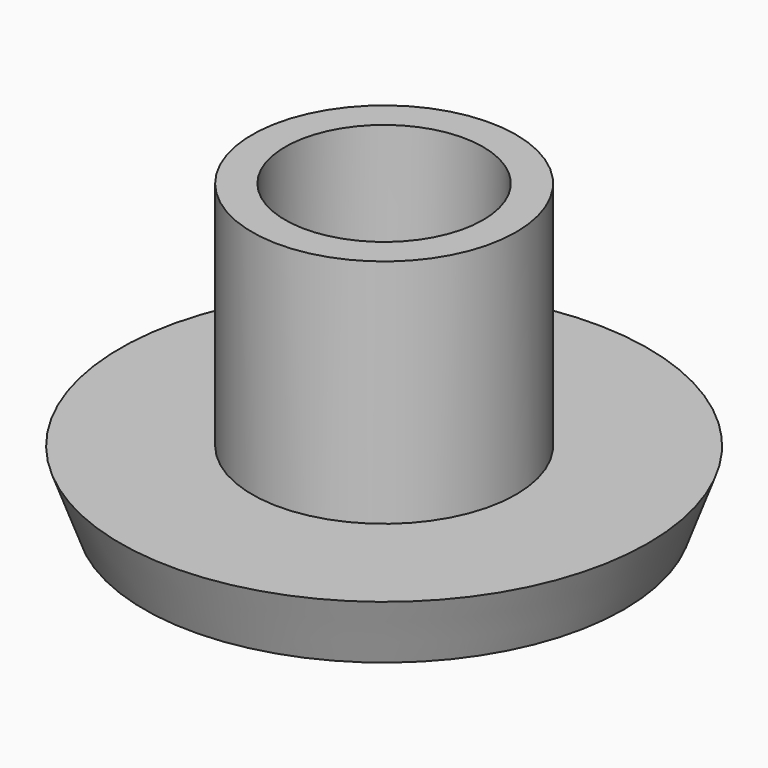
from build123d import *

# Parameters (mm, degrees)
F0_R     = 4
F0_R_2   = 3
F1_DEPTH = 7
F0_R_3   = 8
F2_DEPTH = 2
F3_SIZE2 = 0.72793
F3_SIZE  = 1.99999
F4_DEPTH = 2


# Not quite as in the source:
# - a fillet or chamfer is up to 0.001 mm smaller than in the source, because OpenCascade refuses the exact size


with BuildPart() as f1:
    # F0 (on Top) → F1 (new body)
    with BuildSketch(Plane.XY):
        Circle(F0_R)
        Circle(F0_R_2, mode=Mode.SUBTRACT)
    extrude(amount=F1_DEPTH)


with BuildPart() as f2:
    # F0 (on Top) → F2 (new body)
    with BuildSketch(Plane.XY):
        Circle(F0_R_3)
        Circle(F0_R, mode=Mode.SUBTRACT)
    extrude(amount=-F2_DEPTH)

    # F3 (size 2 and 0.7279404685 in the source; OpenCascade refuses exactly that, so slightly less here)
    f3_edges = [f2.edges().sort_by_distance(p)[0] for p in [
        (-8, 0, -2),
    ]]
    f3_side = f2.faces().sort_by_distance((-8, 0, -1))[0]
    chamfer(f3_edges, length=F3_SIZE, length2=F3_SIZE2, reference=f3_side)


with BuildPart() as f4:
    # F4 (new): a face of the model
    f4_faces = [f1.part.faces().sort_by_distance(p)[0] for p in [
        (-3.886862915, 0, 0),
    ]]
    extrude(f4_faces, amount=F4_DEPTH)


solid = Compound([f1.part, f2.part, f4.part])
